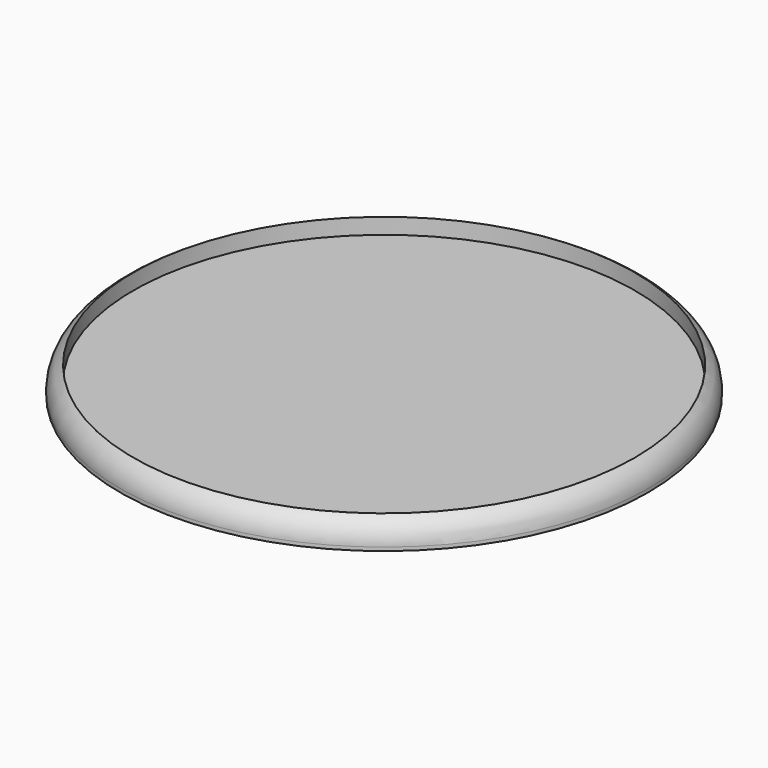
from build123d import *

# Parameters (mm, degrees)
F0_R     = 50
F0_R_2   = 47.5
F1_DEPTH = 5
F3_DEPTH = 2


# Not quite as in the source:
# - a fillet or chamfer that OpenCascade refuses, or shapes differently, is made with other operations: its cross-section is extruded or revolved along the edge and cut away or added


with BuildPart() as f1:
    # F0 (on Top) → F1 (new body)
    with BuildSketch(Plane.XY):
        Circle(F0_R)
        Circle(F0_R_2, mode=Mode.SUBTRACT)
    extrude(amount=F1_DEPTH)

    # F2: fillet of radius 5 on 1 edges, made by hand

    # F2_s1 → F2_t2 (revolve, cut)
    with BuildSketch(Plane.XZ):
        with BuildLine():
            ThreePointArc((50, 0.6698729811), (49.3301270189, 3.1698729811), (47.5, 5))
            Line((47.5, 5), (50, 5))
            Line((50, 5), (50, 0.6698729811))
        make_face()
    revolve(axis=Axis((0, 0, 5), (0, 0, 1)), mode=Mode.SUBTRACT)

    # F0 (on Top) → F3 (join)
    with BuildSketch(Plane.XY):
        Circle(F0_R_2)
    extrude(amount=F3_DEPTH)


solid = f1.part
